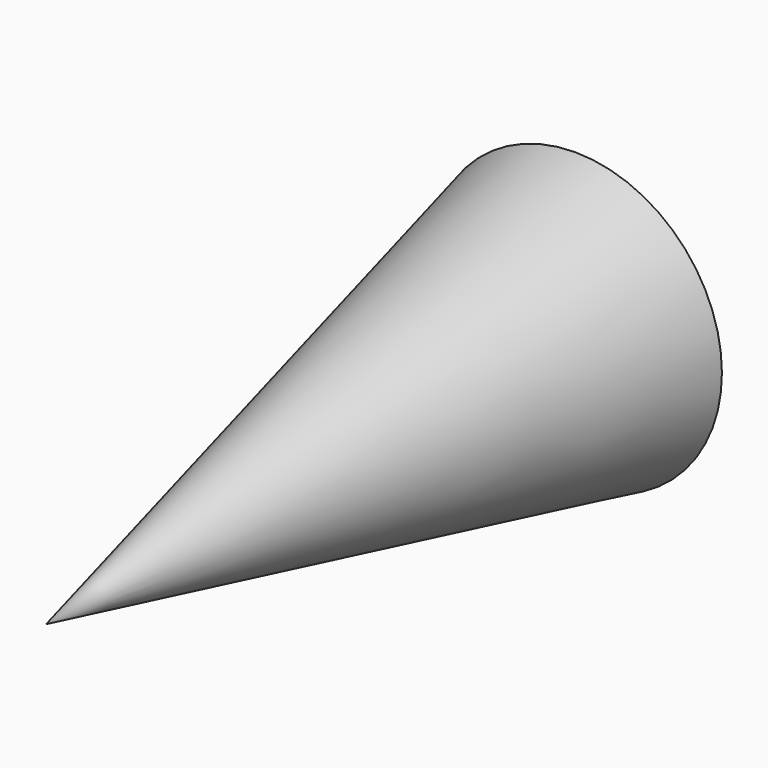
from build123d import *

# Parameters (mm, degrees)
F0_R     = 114.3
F1_DEPTH = 508


# Not quite as in the source:
# - a fillet or chamfer that OpenCascade refuses, or shapes differently, is made with other operations: its cross-section is extruded or revolved along the edge and cut away or added


with BuildPart() as f1:
    # F0 (on Front) → F1 (new body)
    with BuildSketch(Plane.XZ):
        Circle(F0_R)
    extrude(amount=F1_DEPTH)

    # F2: chamfer of 114.3 x 515.5739819686 on 1 edges, made by hand

    # F2_s1 → F2_t2 (revolve, cut)
    with BuildSketch(Plane.XY):
        Polygon((114.3, 7.5739819686), (0, -508), (114.3, -508), align=None)
    revolve(axis=Axis((0, -508, 0), (0, -1, 0)), mode=Mode.SUBTRACT)


solid = f1.part
